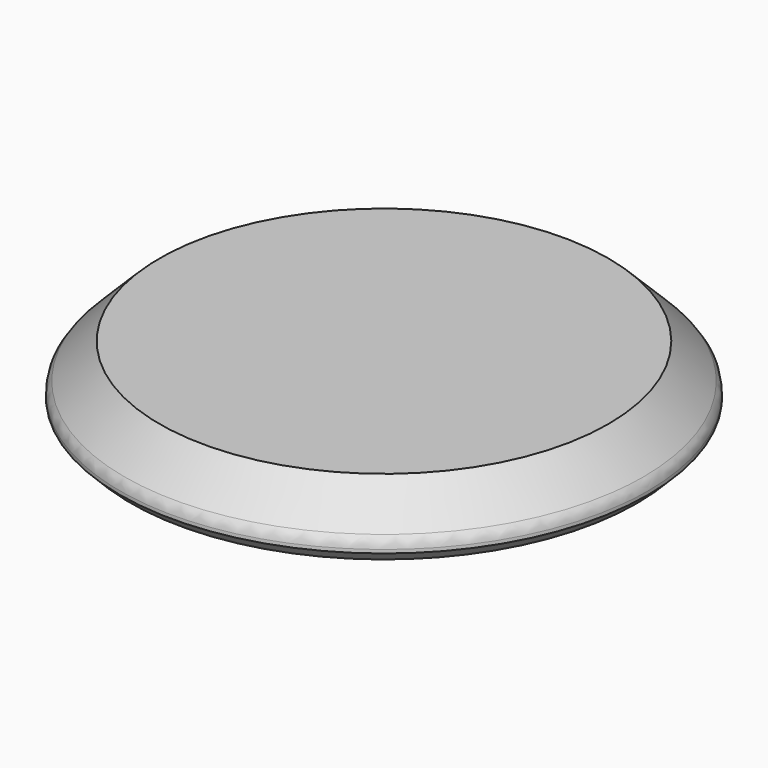
from build123d import *

# Parameters (mm, degrees)
F0_R     = 12
F1_DEPTH = 2.75
F2_R     = 4.02
F3_DEPTH = 4
F4_R     = 6.5
F5_DEPTH = 0.5
F6_SIZE  = 0.49999
F7_SIZE  = 1.8
F8_R     = 0.7


# Not quite as in the source:
# - a fillet or chamfer is up to 0.001 mm smaller than in the source, because OpenCascade refuses the exact size


with BuildPart() as f1:
    # F0 (on Top) → F1 (new body)
    with BuildSketch(Plane.XY):
        Circle(F0_R)
    extrude(amount=F1_DEPTH)

    # F2 (on face) → F3 (join)
    with BuildSketch(Plane(origin=(0, 0, 0), x_dir=(1, 0, 0), z_dir=(0, 0, -1))):
        Circle(F2_R)
    extrude(amount=F3_DEPTH)

    # F4 (on face) → F5 (join)
    with BuildSketch(Plane(origin=(0, 0, 0), x_dir=(1, 0, 0), z_dir=(0, 0, -1))):
        Circle(F4_R)
    extrude(amount=F5_DEPTH)

    # F6 (size 0.5 in the source; OpenCascade refuses exactly that, so slightly less here)
    f6_edges = [f1.edges().sort_by_distance(p)[0] for p in [
        (-6.5, 0, -0.5),
        (-4.02, 0, -4),
        (-12, 0, 0),
    ]]
    chamfer(f6_edges, length=F6_SIZE)

    # F7
    f7_edges = [f1.edges().sort_by_distance(p)[0] for p in [
        (-12, 0, 2.75),
    ]]
    chamfer(f7_edges, length=F7_SIZE)

    # F8
    f8_edges = [f1.edges().sort_by_distance(p)[0] for p in [
        (-12, 0, 0.95),
    ]]
    fillet(f8_edges, radius=F8_R)


solid = f1.part
